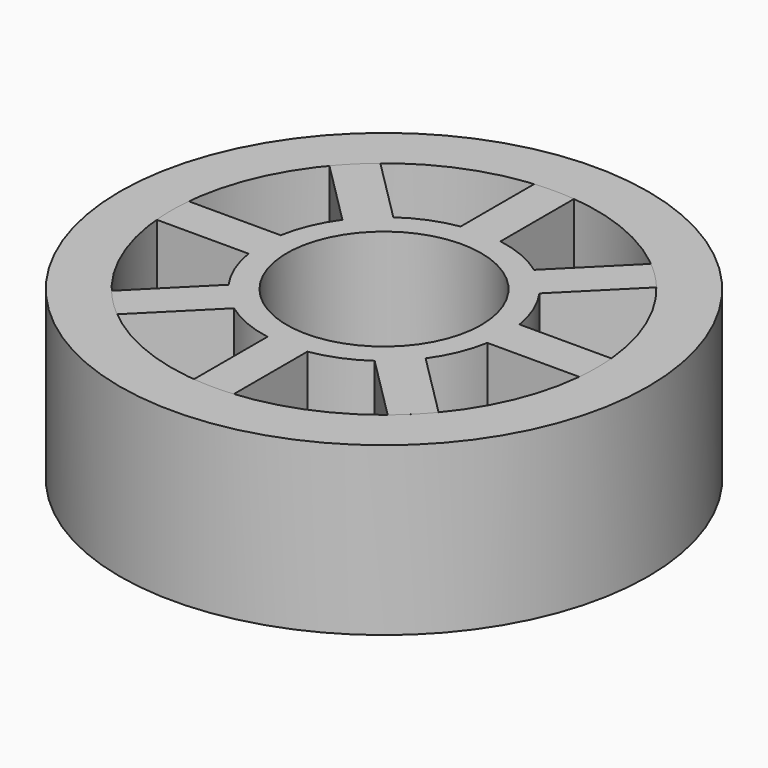
from build123d import *

# Parameters (mm, degrees)
F0_R     = 11.0363
F0_R_2   = 8.89
F1_DEPTH = 6.985
F3_R     = 5.08
F3_R_2   = 4.064
F4_DEPTH = 6.985
F6_DEPTH = 6.985


with BuildPart() as f1:
    # F0 (on Top) → F1 (new body)
    with BuildSketch(Plane.XY):
        Circle(F0_R)
        Circle(F0_R_2, mode=Mode.SUBTRACT)
    extrude(amount=F1_DEPTH)


with BuildPart() as f4:
    # F3 (on face) → F4 (new body)
    with BuildSketch(Plane.XY.offset(6.985)):
        Circle(F3_R)
        Circle(F3_R_2, mode=Mode.SUBTRACT)
    extrude(amount=-F4_DEPTH)

    # F5 (on face) → F6 (join)
    with BuildSketch(Plane.XY.offset(6.985)):
        with BuildLine():
            Line((0, 8.89), (0, 4.588752985))
            Line((0, 4.588752985), (0.8629788063, 4.588752985))
            Line((0.8629788063, 4.588752985), (0.8629788063, 8.8480148949))
            ThreePointArc((0.8629788063, 8.8480148949), (0.4319997596, 8.87949752), (0, 8.89))
        make_face()
        with BuildLine():
            Line((-0.8083467255, 4.6136979945), (0, 4.588752985))
            Line((0, 4.588752985), (0, 8.89))
            ThreePointArc((0, 8.89), (-0.404592586, 8.8807885258), (-0.8083467255, 8.8531731922))
            Line((-0.8083467255, 8.8531731922), (-0.8083467255, 4.6136979945))
        make_face()
        with BuildLine():
            Line((-3.2447383529, 3.2447383529), (-6.2861792847, 6.2861792847))
            ThreePointArc((-6.2861792847, 6.2861792847), (-6.56575595, 5.9935756277), (-6.8317262504, 5.6885513481))
            Line((-6.8317262504, 5.6885513481), (-3.8339645894, 2.6907896871))
            Line((-3.8339645894, 2.6907896871), (-3.2447383529, 3.2447383529))
        make_face()
        with BuildLine():
            Line((-4.588752985, 0.8629788063), (-8.8480148949, 0.8629788063))
            ThreePointArc((-8.8480148949, 0.8629788063), (-8.87949752, 0.4319997596), (-8.89, 0))
            Line((-8.89, 0), (-4.588752985, 0))
            Line((-4.588752985, 0), (-4.588752985, 0.8629788063))
        make_face()
        with BuildLine():
            Line((-4.588752985, 0), (-8.89, 0))
            ThreePointArc((-8.89, 0), (-8.8807885258, -0.404592586), (-8.8531731922, -0.8083467255))
            Line((-8.8531731922, -0.8083467255), (-4.6136979945, -0.8083467255))
            Line((-4.6136979945, -0.8083467255), (-4.588752985, 0))
        make_face()
        with BuildLine():
            Line((-3.8549565188, -2.634520187), (-6.8667094981, -5.6462731663))
            ThreePointArc((-6.8667094981, -5.6462731663), (-6.5842228694, -5.9732829505), (-6.2861792847, -6.2861792847))
            Line((-6.2861792847, -6.2861792847), (-3.2447383529, -3.2447383529))
            Line((-3.2447383529, -3.2447383529), (-3.8549565188, -2.634520187))
        make_face()
        with BuildLine():
            Line((-3.2447383529, -3.2447383529), (-6.2861792847, -6.2861792847))
            ThreePointArc((-6.2861792847, -6.2861792847), (-5.9935756277, -6.56575595), (-5.6885513481, -6.8317262504))
            Line((-5.6885513481, -6.8317262504), (-2.6907896871, -3.8339645894))
            Line((-2.6907896871, -3.8339645894), (-3.2447383529, -3.2447383529))
        make_face()
        with BuildLine():
            Line((-0.8629788063, -4.588752985), (-0.8629788063, -8.8480148949))
            ThreePointArc((-0.8629788063, -8.8480148949), (-0.4319997596, -8.87949752), (0, -8.89))
            Line((0, -8.89), (0, -4.588752985))
            Line((0, -4.588752985), (-0.8629788063, -4.588752985))
        make_face()
        with BuildLine():
            ThreePointArc((0, -8.89), (0.404592586, -8.8807885258), (0.8083467255, -8.8531731922))
            Line((0.8083467255, -8.8531731922), (0.8083467255, -4.6136979945))
            Line((0.8083467255, -4.6136979945), (0, -4.588752985))
            Line((0, -4.588752985), (0, -8.89))
        make_face()
        with BuildLine():
            ThreePointArc((5.6462731663, -6.8667094981), (5.9732829505, -6.5842228694), (6.2861792847, -6.2861792847))
            Line((6.2861792847, -6.2861792847), (3.2447383529, -3.2447383529))
            Line((3.2447383529, -3.2447383529), (2.634520187, -3.8549565188))
            Line((2.634520187, -3.8549565188), (5.6462731663, -6.8667094981))
        make_face()
        with BuildLine():
            ThreePointArc((6.2861792847, -6.2861792847), (6.56575595, -5.9935756277), (6.8317262504, -5.6885513481))
            Line((6.8317262504, -5.6885513481), (3.8339645894, -2.6907896871))
            Line((3.8339645894, -2.6907896871), (3.2447383529, -3.2447383529))
            Line((3.2447383529, -3.2447383529), (6.2861792847, -6.2861792847))
        make_face()
        with BuildLine():
            ThreePointArc((8.8480148949, -0.8629788063), (8.87949752, -0.4319997596), (8.89, 0))
            Line((8.89, 0), (4.588752985, 0))
            Line((4.588752985, 0), (4.588752985, -0.8629788063))
            Line((4.588752985, -0.8629788063), (8.8480148949, -0.8629788063))
        make_face()
        with BuildLine():
            ThreePointArc((8.89, 0), (8.8807885258, 0.404592586), (8.8531731922, 0.8083467255))
            Line((8.8531731922, 0.8083467255), (4.6136979945, 0.8083467255))
            Line((4.6136979945, 0.8083467255), (4.588752985, 0))
            Line((4.588752985, 0), (8.89, 0))
        make_face()
        with BuildLine():
            ThreePointArc((6.8667094981, 5.6462731663), (6.5842228694, 5.9732829505), (6.2861792847, 6.2861792847))
            Line((6.2861792847, 6.2861792847), (3.2447383529, 3.2447383529))
            Line((3.2447383529, 3.2447383529), (3.8549565188, 2.634520187))
            Line((3.8549565188, 2.634520187), (6.8667094981, 5.6462731663))
        make_face()
        with BuildLine():
            ThreePointArc((6.2861792847, 6.2861792847), (5.9935756277, 6.56575595), (5.6885513481, 6.8317262504))
            Line((5.6885513481, 6.8317262504), (2.6907896871, 3.8339645894))
            Line((2.6907896871, 3.8339645894), (3.2447383529, 3.2447383529))
            Line((3.2447383529, 3.2447383529), (6.2861792847, 6.2861792847))
        make_face()
        with BuildLine():
            Line((-2.634520187, 3.8549565188), (-5.6462731663, 6.8667094981))
            ThreePointArc((-5.6462731663, 6.8667094981), (-5.9732829505, 6.5842228694), (-6.2861792847, 6.2861792847))
            Line((-6.2861792847, 6.2861792847), (-3.2447383529, 3.2447383529))
            Line((-3.2447383529, 3.2447383529), (-2.634520187, 3.8549565188))
        make_face()
    extrude(amount=-F6_DEPTH)


solid = Compound([f1.part, f4.part])
